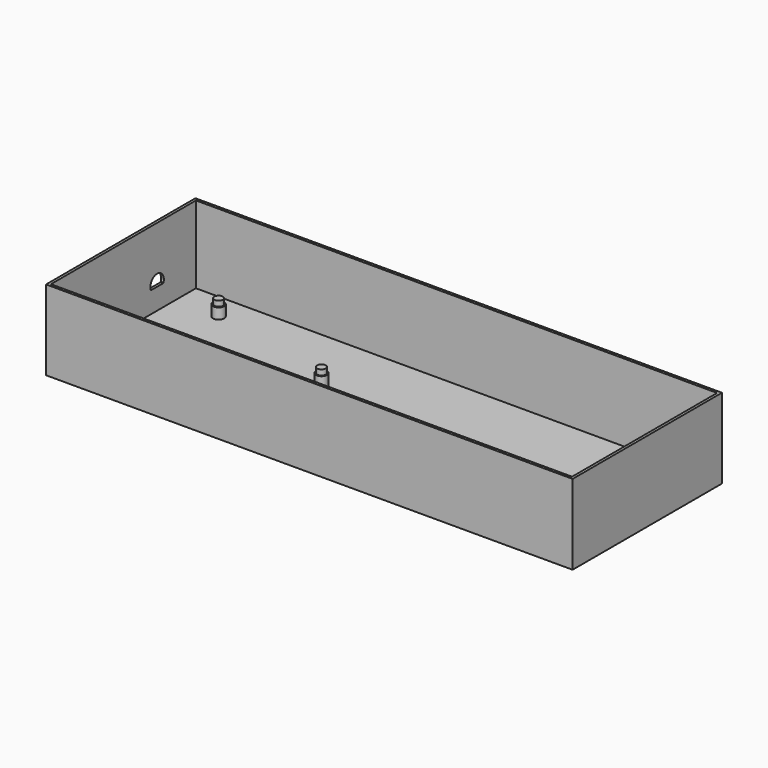
from build123d import *

# Parameters (mm, degrees)
F2_W     = 195.4786418714
F2_H     = 68
F2_R     = 2.1080985417
F2_R_2   = 2.1080985448
F2_R_3   = 2.1080987473
F2_R_4   = 2.1080985484
F3_DEPTH = 1
F2_R_5   = 1.6080985484
F2_R_6   = 1.6080987473
F2_R_7   = 1.6080985448
F2_R_8   = 1.6080985417
F4_DEPTH = 5
F5_DEPTH = 7
F2_H_2   = 1
F2_W_2   = 1
F6_DEPTH = 30
F8_DEPTH = 1


with BuildPart() as f3:
    # F2 (on Top) → F3 (new body)
    with BuildSketch(Plane.XY):
        with Locations((101.2606790643, 35)):
            Rectangle(F2_W, F2_H)
        with Locations((18.551614222, 11.0404381331)):
            Circle(F2_R, mode=Mode.SUBTRACT)
        with Locations((70.5820634049, 16.1186437591)):
            Circle(F2_R_2, mode=Mode.SUBTRACT)
        with Locations((70.5820629074, 44.0276153146)):
            Circle(F2_R_3, mode=Mode.SUBTRACT)
        with Locations((19.8211650697, 59.2622312398)):
            Circle(F2_R_4, mode=Mode.SUBTRACT)
    extrude(amount=F3_DEPTH)

    # F2 (on Top) → F4 (join)
    with BuildSketch(Plane.XY):
        with Locations((19.8211650697, 59.2622312398)):
            Circle(F2_R_4)
        with Locations((19.8211650697, 59.2622312398)):
            Circle(F2_R_5, mode=Mode.SUBTRACT)
        with Locations((70.5820629074, 44.0276153146)):
            Circle(F2_R_3)
        with Locations((70.5820629074, 44.0276153146)):
            Circle(F2_R_6, mode=Mode.SUBTRACT)
        with Locations((70.5820634049, 16.1186437591)):
            Circle(F2_R_2)
        with Locations((70.5820634049, 16.1186437591)):
            Circle(F2_R_7, mode=Mode.SUBTRACT)
        with Locations((18.551614222, 11.0404381331)):
            Circle(F2_R)
        with Locations((18.551614222, 11.0404381331)):
            Circle(F2_R_8, mode=Mode.SUBTRACT)
    extrude(amount=F4_DEPTH)

    # F2 (on Top) → F5 (join)
    with BuildSketch(Plane.XY):
        with Locations((19.8211650697, 59.2622312398)):
            Circle(F2_R_5)
        with Locations((70.5820629074, 44.0276153146)):
            Circle(F2_R_6)
        with Locations((70.5820634049, 16.1186437591)):
            Circle(F2_R_7)
        with Locations((18.551614222, 11.0404381331)):
            Circle(F2_R_8)
    extrude(amount=F5_DEPTH)

    # F2 (on Top) → F6 (join)
    with BuildSketch(Plane.XY):
        with Locations((101.2606790643, 69.5)):
            Rectangle(F2_W, F2_H_2)
        with Locations((199.5, 69.5)):
            Rectangle(F2_W_2, F2_H_2)
        Polygon((2.5213581286, 0), (3.5213581286, 0), (3.5213581286, 1), (3.5213581286, 69), (3.5213581286, 70), (2.5213581286, 70), align=None)
        with Locations((101.2606790643, 0.5)):
            Rectangle(F2_W, F2_H_2)
        with Locations((199.5, 0.5)):
            Rectangle(F2_W_2, F2_H_2)
        with Locations((199.5, 35)):
            Rectangle(F2_W_2, F2_H)
    extrude(amount=F6_DEPTH)

    # F7 (on face) → F8 (cut)
    with BuildSketch(Plane(origin=(2.5213581286, 0, 0), x_dir=(0, -1, 0), z_dir=(-1, 0, 0))):
        with BuildLine():
            Line((-53.966367571, 10.121377154), (-53.966367571, 9.9484939128))
            ThreePointArc((-53.966367571, 9.9484939128), (-53.9072548267, 9.4201302724), (-53.760526233, 8.9091183618))
            Line((-53.760526233, 8.9091183618), (-47.8451862662, 8.9091183618))
            ThreePointArc((-47.8451862662, 8.9091183618), (-47.6903499572, 9.4625889476), (-47.638164158, 10.0349355334))
            ThreePointArc((-47.638164158, 10.0349355334), (-50.7596314072, 13.1993324187), (-53.966367571, 10.121377154))
        make_face()
    extrude(amount=-F8_DEPTH, mode=Mode.SUBTRACT)


solid = f3.part
